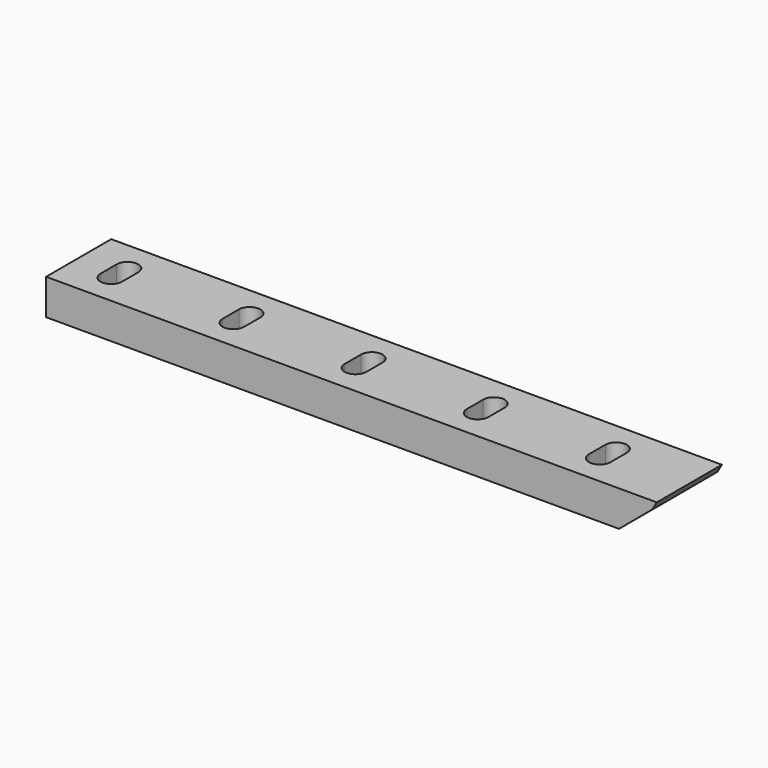
from build123d import *

# Parameters (mm, degrees)
F1_DEPTH = 50.8
F3_DEPTH = 44.451
F4_DEPTH = 25.4


# Not quite as in the source:
# - ends of sketch curves that miss each other by under 0.0002 mm in the source are joined


with BuildPart() as f1:
    # F0 (on Front) → F1 (new body, symmetric)
    with BuildSketch(Plane.XZ):
        Polygon((-347.7068640215, -34.8248227949), (-347.7068640215, -79.2748227949), (367.1742644244, -79.272822397), (408.7938746644, -44.3498227949), (414.2931359785, -34.8248227949), align=None)
    extrude(amount=F1_DEPTH, both=True)

    # F2 (on face) → F3 (cut, through all)
    with BuildSketch(Plane.XY.offset(-34.8248227949)):
        with BuildLine():
            ThreePointArc((-304.0188640215, -12.7), (-296.9068640215, -19.812), (-289.7948640215, -12.7))
            Line((-289.7948640215, -12.7), (-289.7948640215, 12.7))
            ThreePointArc((-289.7948640215, 12.7), (-296.9068640215, 19.812), (-304.0188640215, 12.7))
            Line((-304.0188640215, 12.7), (-304.0188640215, -12.7))
        make_face()
        with BuildLine():
            ThreePointArc((-151.6188640215, -12.7), (-144.5068640215, -19.812), (-137.3948640215, -12.7))
            Line((-137.3948640215, -12.7), (-137.3948640215, 12.7))
            ThreePointArc((-137.3948640215, 12.7), (-144.5068640215, 19.812), (-151.6188640215, 12.7))
            Line((-151.6188640215, 12.7), (-151.6188640215, -12.7))
        make_face()
        with BuildLine():
            ThreePointArc((0.7811359785, -12.7), (7.8931359785, -19.812), (15.0051359785, -12.7))
            Line((15.0051359785, -12.7), (15.0051359785, 12.7))
            ThreePointArc((15.0051359785, 12.7), (7.8931359785, 19.812), (0.7811359785, 12.7))
            Line((0.7811359785, 12.7), (0.7811359785, -12.7))
        make_face()
        with BuildLine():
            ThreePointArc((153.1811359785, -12.7), (160.2931359785, -19.812), (167.4051359785, -12.7))
            Line((167.4051359785, -12.7), (167.4051359785, 12.7))
            ThreePointArc((167.4051359785, 12.7), (160.2931359785, 19.812), (153.1811359785, 12.7))
            Line((153.1811359785, 12.7), (153.1811359785, -12.7))
        make_face()
        with BuildLine():
            ThreePointArc((305.5811359785, -12.7), (312.6931359785, -19.812), (319.8051359785, -12.7))
            Line((319.8051359785, -12.7), (319.8051359785, 12.7))
            ThreePointArc((319.8051359785, 12.7), (312.6931359785, 19.812), (305.5811359785, 12.7))
            Line((305.5811359785, 12.7), (305.5811359785, -12.7))
        make_face()
    extrude(amount=-F3_DEPTH, mode=Mode.SUBTRACT)

    # F2 (on face) → F4 (cut)
    with BuildSketch(Plane.XY.offset(-34.8248227949)):
        with BuildLine():
            ThreePointArc((-283.4448517417, 12.7), (-296.9068640215, 26.1620122798), (-310.3688763013, 12.7))
            Line((-310.3688763013, 12.7), (-310.3688640215, -12.7))
            ThreePointArc((-310.3688640215, -12.7), (-296.9068640215, -26.162), (-283.4448640215, -12.7))
            Line((-283.4448640215, -12.7), (-283.4448517417, 12.7))
        make_face()
        with BuildLine():
            Line((-289.7948640215, 12.7), (-289.7948640215, -12.7))
            ThreePointArc((-289.7948640215, -12.7), (-296.9068640215, -19.812), (-304.0188640215, -12.7))
            Line((-304.0188640215, -12.7), (-304.0188640215, 12.7))
            ThreePointArc((-304.0188640215, 12.7), (-296.9068640215, 19.812), (-289.7948640215, 12.7))
        make_face(mode=Mode.SUBTRACT)
        with BuildLine():
            Line((-157.9688640215, 12.7), (-157.9688640215, -12.7))
            ThreePointArc((-157.9688640215, -12.7), (-144.5068640215, -26.162), (-131.0448640215, -12.7))
            Line((-131.0448640215, -12.7), (-131.0448516369, 12.7))
            ThreePointArc((-131.0448516369, 12.7), (-144.5068640215, 26.1620122798), (-157.9688640215, 12.7))
        make_face()
        with BuildLine():
            Line((-137.3948640215, 12.7), (-137.3948640215, -12.7))
            ThreePointArc((-137.3948640215, -12.7), (-144.5068640215, -19.812), (-151.6188640215, -12.7))
            Line((-151.6188640215, -12.7), (-151.6188640215, 12.7))
            ThreePointArc((-151.6188640215, 12.7), (-144.5068640215, 19.812), (-137.3948640215, 12.7))
        make_face(mode=Mode.SUBTRACT)
        with BuildLine():
            Line((-5.5688640215, 12.7), (-5.5688640215, -12.7))
            ThreePointArc((-5.5688640215, -12.7), (7.8931359785, -26.162), (21.3551359785, -12.7))
            Line((21.3551359785, -12.7), (21.3551483631, 12.7))
            ThreePointArc((21.3551483631, 12.7), (7.8931359785, 26.1620122798), (-5.5688640215, 12.7))
        make_face()
        with BuildLine():
            Line((15.0051359785, 12.7), (15.0051359785, -12.7))
            ThreePointArc((15.0051359785, -12.7), (7.8931359785, -19.812), (0.7811359785, -12.7))
            Line((0.7811359785, -12.7), (0.7811359785, 12.7))
            ThreePointArc((0.7811359785, 12.7), (7.8931359785, 19.812), (15.0051359785, 12.7))
        make_face(mode=Mode.SUBTRACT)
        with BuildLine():
            Line((146.8311359785, 12.7), (146.8311359785, -12.7))
            ThreePointArc((146.8311359785, -12.7), (160.2931359785, -26.162), (173.7551359785, -12.7))
            Line((173.7551359785, -12.7), (173.7551483631, 12.7))
            ThreePointArc((173.7551483631, 12.7), (160.2931359785, 26.1620122798), (146.8311359785, 12.7))
        make_face()
        with BuildLine():
            Line((167.4051359785, 12.7), (167.4051359785, -12.7))
            ThreePointArc((167.4051359785, -12.7), (160.2931359785, -19.812), (153.1811359785, -12.7))
            Line((153.1811359785, -12.7), (153.1811359785, 12.7))
            ThreePointArc((153.1811359785, 12.7), (160.2931359785, 19.812), (167.4051359785, 12.7))
        make_face(mode=Mode.SUBTRACT)
        with BuildLine():
            Line((299.2311359785, 12.7), (299.2311359785, -12.7))
            ThreePointArc((299.2311359785, -12.7), (312.6931359785, -26.162), (326.1551359785, -12.7))
            Line((326.1551359785, -12.7), (326.1551483631, 12.7))
            ThreePointArc((326.1551483631, 12.7), (312.6931359785, 26.1620122798), (299.2311359785, 12.7))
        make_face()
        with BuildLine():
            Line((319.8051359785, 12.7), (319.8051359785, -12.7))
            ThreePointArc((319.8051359785, -12.7), (312.6931359785, -19.812), (305.5811359785, -12.7))
            Line((305.5811359785, -12.7), (305.5811359785, 12.7))
            ThreePointArc((305.5811359785, 12.7), (312.6931359785, 19.812), (319.8051359785, 12.7))
        make_face(mode=Mode.SUBTRACT)
    extrude(amount=-F4_DEPTH, mode=Mode.SUBTRACT)


solid = f1.part
